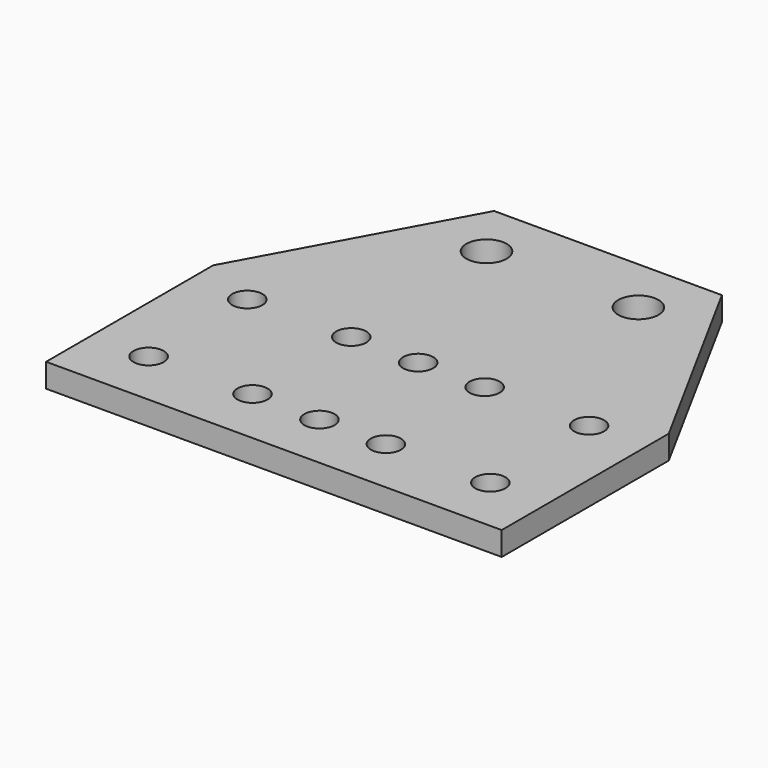
from build123d import *

# Parameters (mm, degrees)
F0_W     = 19.05
F0_H     = 19.05
F0_W_2   = 12.7
F1_DEPTH = 7.9375
F2_D     = 10.0838
F3_D     = 13.49248


# Not quite as in the source:
# - a feature names something its author has since deleted; it is built from what else it names


with BuildPart() as f1:
    # F0 (on Top) → F1 (new body)
    with BuildSketch(Plane.XY):
        with Locations((-66.5298237595, -51.1898304701)):
            Rectangle(F0_W, F0_H)
        Polygon((-57.0048237595, -41.6648304701), (-57.0048237595, -60.7148304701), (-37.9548237595, -60.7148304701), (-37.9548237595, 9.1351695299), (-76.0548237595, 9.1351695299), (-76.0548237595, -41.6648304701), align=None)
        Polygon((-37.9548237595, 9.1351695299), (-37.9548237595, -60.7148304701), (0.1451762405, -60.7148304701), (0.1451762405, -41.6648304701), (0.1451762405, -0.3898304701), (22.3701762405, -0.3898304701), (22.3701762405, -41.6648304701), (22.3701762405, -60.7148304701), (38.2451762405, -60.7148304701), (38.2451762405, 9.1351695299), align=None)
        Polygon((-37.9548237595, 78.9851695299), (-76.0548237595, 9.1351695299), (-37.9548237595, 9.1351695299), (-37.9548237595, 59.9351695299), align=None)
        Polygon((0.1451762405, -41.6648304701), (0.1451762405, -60.7148304701), (22.3701762405, -60.7148304701), (22.3701762405, -41.6648304701), (22.3701762405, -0.3898304701), (0.1451762405, -0.3898304701), align=None)
        Polygon((-37.9548237595, 59.9351695299), (-37.9548237595, 9.1351695299), (38.2451762405, 9.1351695299), (38.2451762405, 59.9351695299), (25.5451762405, 59.9351695299), (25.5451762405, 78.9851695299), (-25.2548237595, 78.9851695299), (-25.2548237595, 59.9351695299), align=None)
        with Locations((-31.6048237595, 69.4601695299)):
            Rectangle(F0_W_2, F0_H)
        Polygon((38.2451762405, 59.9351695299), (38.2451762405, 9.1351695299), (76.3451762405, 9.1351695299), (38.2451762405, 78.9851695299), align=None)
        Polygon((76.3451762405, 9.1351695299), (38.2451762405, 9.1351695299), (38.2451762405, -60.7148304701), (57.2951762405, -60.7148304701), (76.3451762405, -60.7148304701), align=None)
        with Locations((31.8951762405, 69.4601695299)):
            Rectangle(F0_W_2, F0_H)
    extrude(amount=F1_DEPTH)

    # F2 (through all)
    with Locations(Plane(origin=(0, 0, 0), x_dir=(1, 0, 0), z_dir=(0, 0, -1))):
        with Locations((-57.0048237595, 0.3898304701), (-57.0048237595, 41.6648304701), (0.1451762405, 0.3898304701), (0.1451762405, 41.6648304701), (57.2951762405, 0.3898304701), (57.2951762405, 41.6648304701), (-22.5665104002, 0), (-22.5665104002, 41.275), (22.3701762405, 41.6648304701), (22.3701762405, 0.3898304701)):
            Hole(F2_D / 2)

    # F3 (through all)
    with Locations(Plane(origin=(0, 0, 0), x_dir=(1, 0, 0), z_dir=(0, 0, -1))):
        with Locations((-25.2548237595, -59.9351695299), (25.5451762405, -59.9351695299)):
            Hole(F3_D / 2)


solid = f1.part
